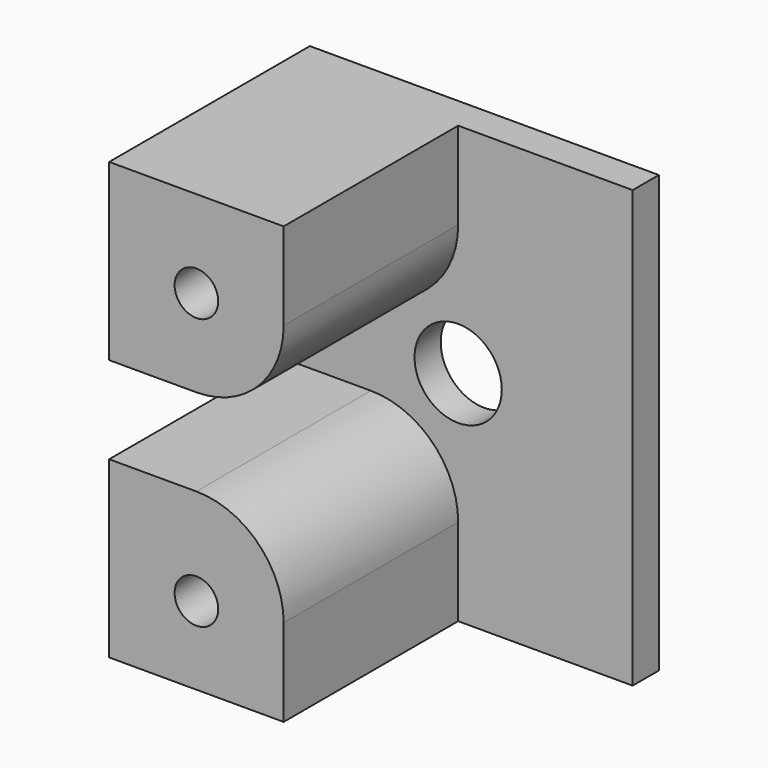
from build123d import *

# Parameters (mm, degrees)
F0_W        = 101.6
F0_H        = 127
F1_DEPTH    = 9.525
F2_R        = 12.7
F3_DEPTH    = 63.5
F4_W        = 50.8
F4_H        = 50.8
F5_DEPTH    = 63.5
F6_W        = 50.8
F6_H        = 50.8
F7_DEPTH    = 63.5
F8_T1_DEPTH = 127
F9_R        = 25.4
F10_R       = 6.35
F11_DEPTH   = 12.7
F12_R       = 6.35
F13_DEPTH   = 12.7


# Not quite as in the source:
# - a fillet or chamfer that OpenCascade refuses, or shapes differently, is made with other operations: its cross-section is extruded or revolved along the edge and cut away or added


with BuildPart() as f1:
    # F0 (on Front) → F1 (new body)
    with BuildSketch(Plane.XZ):
        Rectangle(F0_W, F0_H)
    extrude(amount=F1_DEPTH)

    # F2 (on face) → F3 (cut)
    with BuildSketch(Plane.XZ.offset(9.525)):
        Circle(F2_R)
    extrude(amount=-F3_DEPTH, mode=Mode.SUBTRACT)

    # F4 (on face) → F5 (join)
    with BuildSketch(Plane.XZ.offset(9.525)):
        with Locations((-25.4, -38.1)):
            Rectangle(F4_W, F4_H)
    extrude(amount=F5_DEPTH)

    # F6 (on face) → F7 (join)
    with BuildSketch(Plane.XZ.offset(9.525)):
        with Locations((-25.4, 38.1)):
            Rectangle(F6_W, F6_H)
    extrude(amount=F7_DEPTH)

    # F8: fillet of radius 25.4 on 1 edges, made by hand

    # F8_s2 → F8_t1 (cut)
    with BuildSketch(Plane.XZ.offset(9.525)):
        with BuildLine():
            ThreePointArc((-25.4, -12.7), (-7.4394877579, -20.1394877579), (0, -38.1))
            Line((0, -38.1), (0, -12.7))
            Line((0, -12.7), (-25.4, -12.7))
        make_face()
    extrude(amount=F8_T1_DEPTH, mode=Mode.SUBTRACT)

    # F9
    f9_edges = [f1.edges().sort_by_distance(p)[0] for p in [
        (0, -41.275, 12.7),
    ]]
    fillet(f9_edges, radius=F9_R)

    # F10 (on face) → F11 (cut)
    with BuildSketch(Plane.XZ.offset(73.025)):
        with Locations((-25.4, -40.7783836126)):
            Circle(F10_R)
    extrude(amount=-F11_DEPTH, mode=Mode.SUBTRACT)

    # F12 (on face) → F13 (cut)
    with BuildSketch(Plane.XZ.offset(73.025)):
        with Locations((-25.4, 38.1)):
            Circle(F12_R)
    extrude(amount=-F13_DEPTH, mode=Mode.SUBTRACT)


solid = f1.part
